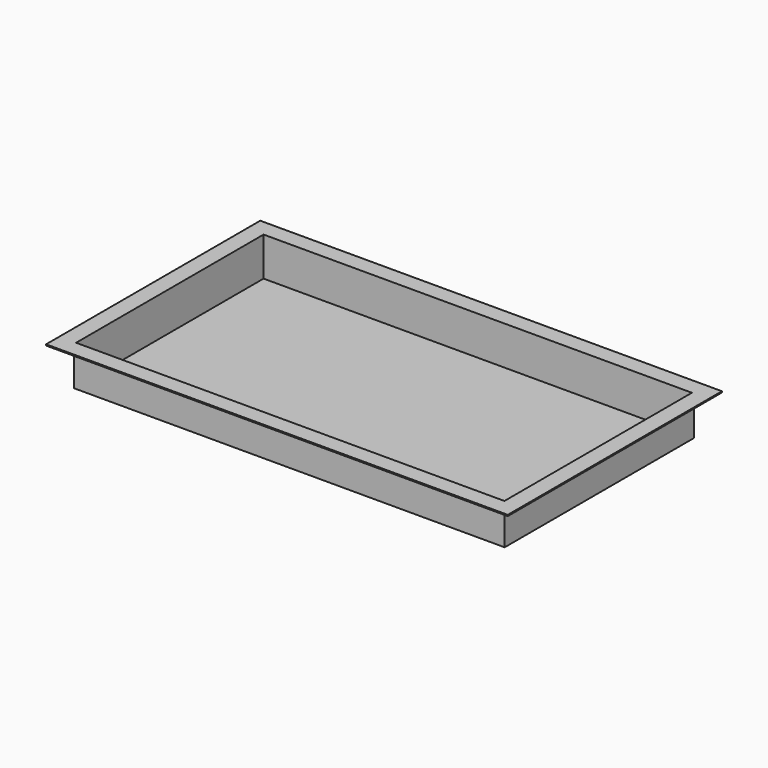
from build123d import *

# Parameters (mm, degrees)
F0_W        = 555
F0_H        = 305
F1_DEPTH    = 50
F2_W        = 595
F2_H        = 345
F2_W_2      = 555
F2_H_2      = 305
F3_DEPTH    = 1.5
F4_T        = 1.5
F4_T3_DEPTH = 308
F4_T5_DEPTH = 558


# Not quite as in the source:
# - a shell that OpenCascade refuses in one call is made with other operations: the cavity is built on its own and cut out


with BuildPart() as f1:
    # F0 (on Top) → F1 (new body)
    with BuildSketch(Plane.XY):
        Rectangle(F0_W, F0_H)
    extrude(amount=-F1_DEPTH)

    # F2 (on face) → F3 (join)
    with BuildSketch(Plane.XY):
        Rectangle(F2_W, F2_H)
        Rectangle(F2_W_2, F2_H_2, mode=Mode.SUBTRACT)
        Rectangle(F2_W_2, F2_H_2)
    extrude(amount=F3_DEPTH)

    # F4: shell of thickness 1.5, made by hand


with BuildPart() as f4_core1:
    # F4_t2: copy of F1
    add(f1.part)

    # the walls: a layer under each face that stays
    f4_faces = [f4_core1.faces().sort_by_distance(p)[0] for p in [
        (-297.5, 0, 0.75),
        (0, 172.5, 0.75),
        (0, -172.5, 0.75),
        (-277.6666666667, -161, 0),
        (297.5, 0, 0.75),
        (-277.5, 0, -25),
        (0, -152.5, -25),
        (277.5, 0, -25),
        (0, 152.5, -25),
        (0, 0, -50),
    ]]
    thicken(f4_faces, amount=-F4_T, mode=Mode.SUBTRACT)

    # F4_s4 → F4_t3 (cut)
    with BuildSketch(Plane.XZ.offset(-154)):
        Polygon((-277.515, -0.015), (-277.5, 1.5), (-276, 1.5), (-276, 0), align=None)
        Polygon((277.515, -0.015), (277.5, 1.5), (276, 1.5), (276, 0), align=None)
    extrude(amount=F4_T3_DEPTH, mode=Mode.SUBTRACT)

    # F4_s6 → F4_t5 (cut)
    with BuildSketch(Plane.YZ.offset(-279)):
        Polygon((-152.515, -0.015), (-152.5, 1.5), (-151, 1.5), (-151, 0), align=None)
        Polygon((152.515, -0.015), (152.5, 1.5), (151, 1.5), (151, 0), align=None)
    extrude(amount=F4_T5_DEPTH, mode=Mode.SUBTRACT)


with BuildPart() as f1_1:
    add(f1.part)

    # what is left inside the walls is the cavity
    f4_cavity = [f4_core1.part.solids().sort_by_distance(p)[0] for p in [
        (0, -50.333333, -48.485),
    ]]
    add(f4_cavity, mode=Mode.SUBTRACT)


solid = f1_1.part
